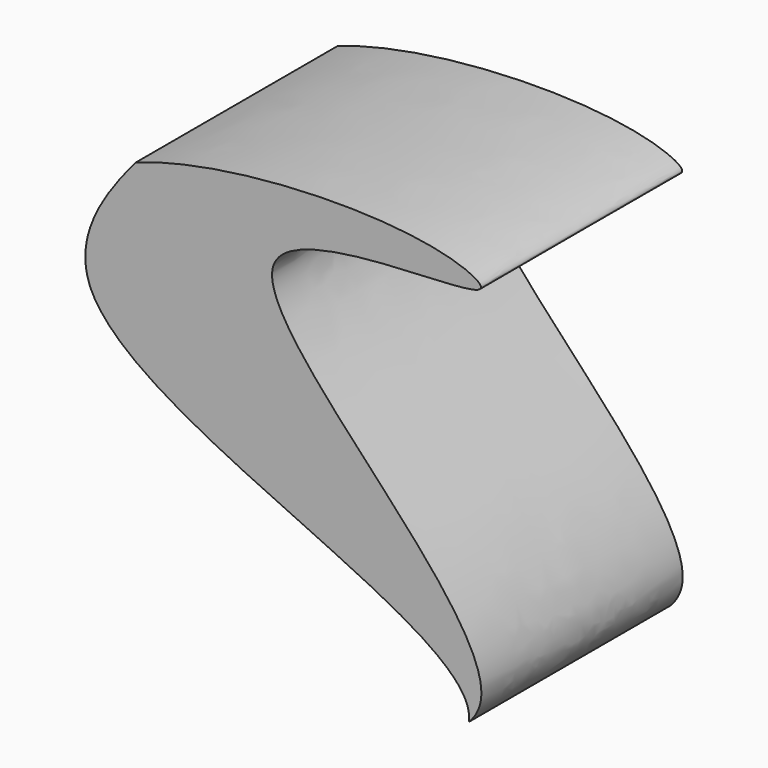
from build123d import *

# Parameters (mm, degrees)
F1_DEPTH = 50.038


with BuildPart() as f1:
    # F0 (on Front) → F1 (new body)
    with BuildSketch(Plane.XZ):
        with BuildLine():
            add(Edge.make_bspline(
                [(79.1851501145, 33.667985141), (75.0187026574, 31.503252156), (-2.4379861385, 37.6481391794), (87.3723170721, -25.341323607), (78.5399634882, -41.3093671709), (77.274699503, -42.6143057432)],
                knots=[0, 0, 0, 0, 0.1298884954, 0.304379438, 0.3223113992, 0.3223113992, 0.3223113992, 0.3223113992], degree=3))
            add(Edge.make_bspline(
                [(11.1058921605, 33.8209956614), (14.4397051782, 35.019855662), (34.6725145866, 40.4657294514), (69.9810109278, 40.6166271778), (80.8246080885, 34.5197872555), (79.1851501145, 33.667985141)],
                knots=[0.771168741, 0.771168741, 0.771168741, 0.771168741, 0.8043873432, 0.948890096, 1, 1, 1, 1], degree=3))
            add(Edge.make_bspline(
                [(1.8684788003, 9.321059509), (-1.3841643437, 17.6719319964), (5.2084741646, 26.9707864304), (11.1058921562, 33.8209956571)],
                knots=[0.5042673301, 0.5042673301, 0.5042673301, 0.5042673301, 0.5962648223, 0.5962648223, 0.5962648223, 0.5962648223], degree=3))
            add(Edge.make_bspline(
                [(2.0611278183, 8.853789435), (1.9972476452, 9.0103169518), (1.9330033894, 9.1660713289), (1.8684788033, 9.3210595026)],
                knots=[0.6304405304, 0.6304405304, 0.6304405304, 0.6304405304, 0.6322791361, 0.6322791361, 0.6322791361, 0.6322791361], degree=3))
            add(Edge.make_bspline(
                [(77.274699503, -42.6143057432), (79.4681300041, -26.5906033467), (11.0260514961, -11.7528920899), (2.0611278183, 8.853789435)],
                knots=[0.2745709496, 0.2745709496, 0.2745709496, 0.2745709496, 0.5025477969, 0.5025477969, 0.5025477969, 0.5025477969], degree=3))
        make_face()
    extrude(amount=F1_DEPTH)


solid = f1.part
